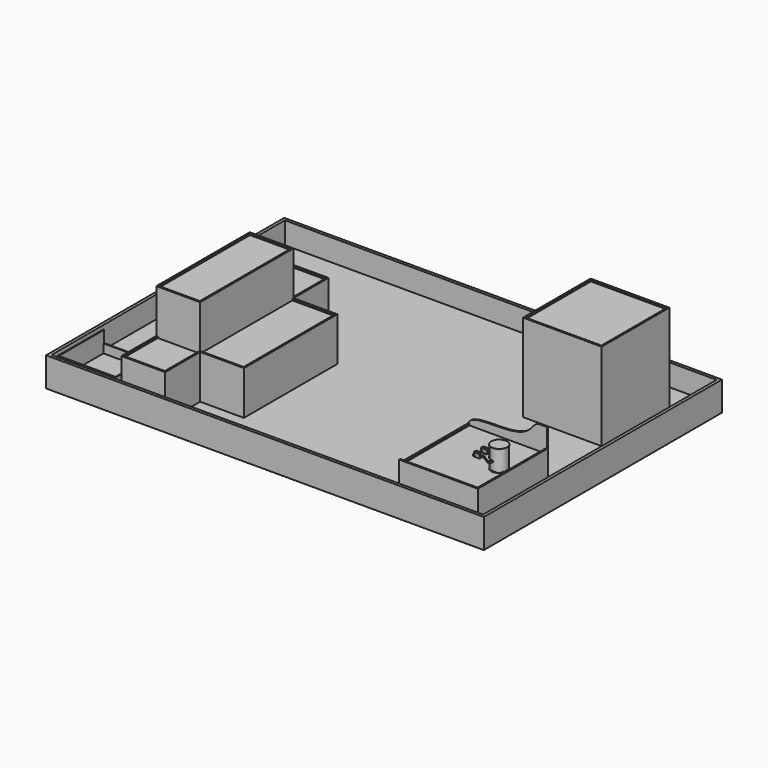
from build123d import *

# Parameters (mm, degrees)
F0_R      = 27.2
F1_DEPTH  = 2.83
F2_R      = 26.4
F3_DEPTH  = 67.36
F4_R      = 27.2
F5_DEPTH  = 2.83
F9_W      = 270
F9_H      = 300
F10_DEPTH = 72
F12_DEPTH = 15
F14_DEPTH = 5
F15_W     = 5
F15_H     = 290
F16_DEPTH = 5
F17_W     = 1500
F17_H     = 1020
F18_DEPTH = 25
F19_W     = 270
F19_H     = 290
F20_DEPTH = 300
F21_W     = 260
F21_H     = 280
F22_DEPTH = 5
F23_W     = 1500
F23_H     = 1020
F23_W_2   = 1480
F23_H_2   = 1000
F24_DEPTH = 75
F26_DEPTH = 150
F27_W     = 150
F27_H     = 400
F28_DEPTH = 150
F29_W     = 140
F29_H     = 390
F30_DEPTH = 5
F31_W     = 140
F31_H     = 145
F31_W_2   = 145
F31_H_2   = 390
F32_DEPTH = 5
F33_R     = 3
F34_DEPTH = 4
F35_R     = 3.99999
F35_2_R   = 3.99999
F36_R     = 3
F37_DEPTH = 8
F38_R     = 3
F39_DEPTH = 8
F40_R     = 3
F40_R_2   = 2.5
F41_DEPTH = 3
F42_R     = 3
F42_R_2   = 2.5
F43_DEPTH = 3
F45_DEPTH = 270.001
F46_W     = 200
F46_H     = 200
F46_W_2   = 194
F46_H_2   = 191
F47_DEPTH = 30
F49_DEPTH = 40
F50_R     = 2.9331626505
F50_R_2   = 2.6879545315
F50_R_3   = 3
F50_R_4   = 2.8111339575
F51_DEPTH = 6


# Not quite as in the source:
# - a fillet or chamfer is up to 0.001 mm smaller than in the source, because OpenCascade refuses the exact size
# - a feature names something its author has since deleted; it is built from what else it names


with BuildPart() as f1:
    # F0 (on Top) → F1 (new body)
    with BuildSketch(Plane.XY):
        Circle(F0_R)
    extrude(amount=F1_DEPTH)

    # F2 (on face) → F3 (join)
    with BuildSketch(Plane.XY.offset(2.83)):
        Circle(F2_R)
    extrude(amount=F3_DEPTH)

    # F4 (on face) → F5 (join)
    with BuildSketch(Plane.XY.offset(70.19)):
        Circle(F4_R)
    extrude(amount=F5_DEPTH)


with BuildPart() as f10:
    # F9 (on Top) → F10 (new body)
    with BuildSketch(Plane.XY):
        with Locations((-87.8, 0)):
            Rectangle(F9_W, F9_H)
    extrude(amount=-F10_DEPTH)

    # F11 (on face) → F12 (join)
    with BuildSketch(Plane.XY):
        Polygon((-222.8, -145), (-222.8, -150), (47.2, -150), (47.2, 150), (42.2, 150), (42.2, -145), align=None)
    extrude(amount=F12_DEPTH)

    # F13 (on face) → F14 (join)
    with BuildSketch(Plane(origin=(0, 150, 0), x_dir=(-1, 0, 0), z_dir=(0, 1, 0))):
        with BuildLine():
            Line((-21.3134280931, 81.3575685024), (-47.2, 81.3575685024))
            Line((-47.2, 81.3575685024), (-47.2, -72))
            Line((-47.2, -72), (222.8, -72))
            Line((222.8, -72), (222.8, 0))
            add(Edge.make_bspline(
                [(-21.3134280931, 81.3575685024), (-6.3059147253, 81.3822787863), (12.9585432644, 38.1268753575), (103.6097013063, 23.6068887567), (223.0224295336, 30.7718731823), (222.8, 0)],
                knots=[0, 0, 0, 0, 0.2487100673, 0.6151112321, 1, 1, 1, 1], degree=3))
        make_face()
    extrude(amount=-F14_DEPTH)

    # F15 (on face) → F16 (join)
    with BuildSketch(Plane.XY):
        with Locations((-220.3, 0)):
            Rectangle(F15_W, F15_H)
    extrude(amount=F16_DEPTH)

    # F17 (on face) → F18 (join)
    with BuildSketch(Plane(origin=(0, 0, -72), x_dir=(1, 0, 0), z_dir=(0, 0, -1))):
        with Locations((-602.8, -260)):
            Rectangle(F17_W, F17_H)
    extrude(amount=F18_DEPTH)

    # F19 (on face) → F20 (join)
    with BuildSketch(Plane.XY.offset(-72)):
        with Locations((-87.8, 525)):
            Rectangle(F19_W, F19_H)
    extrude(amount=F20_DEPTH)

    # F21 (on face) → F22 (cut)
    with BuildSketch(Plane.XY.offset(228)):
        with Locations((-87.8, 525)):
            Rectangle(F21_W, F21_H)
    extrude(amount=-F22_DEPTH, mode=Mode.SUBTRACT)

    # F23 (on face) → F24 (join)
    with BuildSketch(Plane.XY.offset(-72)):
        with Locations((-602.8, 260)):
            Rectangle(F23_W, F23_H)
        with Locations((-602.8, 260)):
            Rectangle(F23_W_2, F23_H_2, mode=Mode.SUBTRACT)
    extrude(amount=F24_DEPTH)

    # F25 (on face) → F26 (join)
    with BuildSketch(Plane.XY.offset(-72)):
        Polygon((-952.8, 460), (-1102.8, 460), (-1102.8, -240), (-952.8, -240), (-952.8, -90), (-802.8, -90), (-802.8, 310), (-952.8, 310), align=None)
    extrude(amount=F26_DEPTH)

    # F27 (on face) → F28 (join)
    with BuildSketch(Plane.XY.offset(78)):
        with Locations((-1027.8, 110)):
            Rectangle(F27_W, F27_H)
    extrude(amount=F28_DEPTH)

    # F29 (on face) → F30 (cut)
    with BuildSketch(Plane.XY.offset(228)):
        with Locations((-1027.8, 110)):
            Rectangle(F29_W, F29_H)
    extrude(amount=-F30_DEPTH, mode=Mode.SUBTRACT)

    # F31 (on face) → F32 (cut)
    with BuildSketch(Plane.XY.offset(78)):
        with Locations((-1027.8, 382.5)):
            Rectangle(F31_W, F31_H)
        with Locations((-880.3, 110)):
            Rectangle(F31_W_2, F31_H_2)
        with Locations((-1027.8, -162.5)):
            Rectangle(F31_W, F31_H)
    extrude(amount=-F32_DEPTH, mode=Mode.SUBTRACT)

    # F46 (on face) → F47 (join)
    with BuildSketch(Plane.XY.offset(-72)):
        with Locations((-1232.8, -130)):
            Rectangle(F46_W, F46_H)
        with Locations((-1232.8, -128.5)):
            Rectangle(F46_W_2, F46_H_2, mode=Mode.SUBTRACT)
    extrude(amount=F47_DEPTH)

    # F48 (on face) → F49 (join)
    with BuildSketch(Plane.XY.offset(-42)):
        Polygon((-1329.8, -30), (-1332.8, -30), (-1332.8, -230), (-1329.8, -230), (-1135.8, -230), (-1132.8, -230), (-1132.8, -30), (-1135.8, -30), (-1135.8, -224), (-1329.8, -224), align=None)
    extrude(amount=F49_DEPTH)


with BuildPart() as f34:
    # F33 (on offset) → F34 (new body, symmetric)
    with BuildSketch(Plane.XY.offset(25)):
        with BuildLine():
            Line((-55, -12), (-74.5, -12))
            Line((-74.5, -12), (-74.5, -13))
            Line((-74.5, -13), (-65.6457513111, -13))
            ThreePointArc((-65.6457513111, -13), (-67, -16), (-65.6457513111, -19))
            Line((-65.6457513111, -19), (-74.5, -19))
            Line((-74.5, -19), (-74.5, -20))
            Line((-74.5, -20), (-55, -20))
            ThreePointArc((-55, -20), (-51, -16), (-55, -12))
        make_face()
        with Locations((-63, -16)):
            Circle(F33_R, mode=Mode.SUBTRACT)
        with Locations((-55, -16)):
            Circle(F33_R, mode=Mode.SUBTRACT)
    extrude(amount=F34_DEPTH, both=True)

    # F35 (radius 4 in the source; OpenCascade refuses exactly that, so slightly less here)
    f35_edges = [f34.edges().sort_by_distance(p)[0] for p in [
        (-74.5, -19.5, 29),
        (-74.5, -12.5, 29),
        (-74.5, -19.5, 21),
        (-74.5, -12.5, 21),
    ]]
    fillet(f35_edges, radius=F35_R)

    # F36 (on face) → F37 (join, through all)
    with BuildSketch(Plane.XZ.offset(20)):
        with Locations((-70.5, 25)):
            Circle(F36_R)
    extrude(amount=-F37_DEPTH)

    # F42 (on offset) → F43 (join, symmetric)
    with BuildSketch(Plane.XY.offset(25)):
        with Locations((-63, -16)):
            Circle(F42_R)
        with Locations((-63, -16)):
            Circle(F42_R_2, mode=Mode.SUBTRACT)
        with Locations((-55, -16)):
            Circle(F42_R)
        with Locations((-55, -16)):
            Circle(F42_R_2, mode=Mode.SUBTRACT)
    extrude(amount=F43_DEPTH, both=True)


with BuildPart() as f34b:
    # F33 (on offset) → F34, piece 2 (new body, symmetric)
    with BuildSketch(Plane.XY.offset(25)):
        with BuildLine():
            Line((-74.5, 13), (-74.5, 12))
            Line((-74.5, 12), (-55, 12))
            ThreePointArc((-55, 12), (-51, 16), (-55, 20))
            Line((-55, 20), (-74.5, 20))
            Line((-74.5, 20), (-74.5, 19))
            Line((-74.5, 19), (-65.6457513111, 19))
            ThreePointArc((-65.6457513111, 19), (-67, 16), (-65.6457513111, 13))
            Line((-65.6457513111, 13), (-74.5, 13))
        make_face()
        with Locations((-63, 16)):
            Circle(F33_R, mode=Mode.SUBTRACT)
        with Locations((-55, 16)):
            Circle(F33_R, mode=Mode.SUBTRACT)
    extrude(amount=F34_DEPTH, both=True)

    # F35#2 (radius 4 in the source; OpenCascade refuses exactly that, so slightly less here)
    f35_2_edges = [f34b.edges().sort_by_distance(p)[0] for p in [
        (-74.5, 12.5, 29),
        (-74.5, 19.5, 29),
        (-74.5, 19.5, 21),
        (-74.5, 12.5, 21),
    ]]
    fillet(f35_2_edges, radius=F35_2_R)

    # F38 (on face) → F39 (join, through all)
    with BuildSketch(Plane(origin=(0, 20, 0), x_dir=(-1, 0, 0), z_dir=(0, 1, 0))):
        with Locations((70.5, 25)):
            Circle(F38_R)
    extrude(amount=-F39_DEPTH)

    # F40 (on offset) → F41 (join, symmetric)
    with BuildSketch(Plane.XY.offset(25)):
        with Locations((-55, 16)):
            Circle(F40_R)
        with Locations((-55, 16)):
            Circle(F40_R_2, mode=Mode.SUBTRACT)
        with Locations((-63, 16)):
            Circle(F40_R)
        with Locations((-63, 16)):
            Circle(F40_R_2, mode=Mode.SUBTRACT)
    extrude(amount=F41_DEPTH, both=True)


with BuildPart() as f45_tool:
    # F44 (on face) → F45 (new body, through all)
    with BuildSketch(Plane(origin=(0, 20, 0), x_dir=(-1, 0, 0), z_dir=(0, 1, 0))):
        with BuildLine():
            Line((71.5, 26), (71.5, 27.2912878475))
            ThreePointArc((71.5, 27.2912878475), (70.5, 27.5), (69.5, 27.2912878475))
            Line((69.5, 27.2912878475), (69.5, 26))
            Line((69.5, 26), (68.2087121525, 26))
            ThreePointArc((68.2087121525, 26), (68, 25), (68.2087121525, 24))
            Line((68.2087121525, 24), (69.5, 24))
            Line((69.5, 24), (69.5, 22.7087121525))
            ThreePointArc((69.5, 22.7087121525), (70.5, 22.5), (71.5, 22.7087121525))
            Line((71.5, 22.7087121525), (71.5, 24))
            Line((71.5, 24), (72.7912878475, 24))
            ThreePointArc((72.7912878475, 24), (73, 25), (72.7912878475, 26))
            Line((72.7912878475, 26), (71.5, 26))
        make_face()
    extrude(amount=-F45_DEPTH)


with BuildPart() as f34_1:
    add(f34.part)

    # F45: cut by f45_tool
    add(f45_tool.part, mode=Mode.SUBTRACT)


with BuildPart() as f34b_1:
    add(f34b.part)

    # F45: cut by f45_tool
    add(f45_tool.part, mode=Mode.SUBTRACT)


with BuildPart() as f51:
    # F50 (on face) → F51 (new body)
    with BuildSketch(Plane.XY.offset(29)):
        with BuildLine():
            ThreePointArc((0.73436121, -28.0007835725), (-28.0000147608, -0.763112347), (-0.7918626795, 27.9992164275))
            Line((-0.7918626795, 27.9992164275), (-5.8697271642, 34.7379657611))
            ThreePointArc((-5.8697271642, 34.7379657611), (-9.0911257385, 36.6690164274), (-12.7480278467, 35.812609736))
            Line((-12.7480278467, 35.812609736), (-33.2897768634, 21.3))
            Line((-33.2897768634, 21.3), (-68.6539217851, 21.3))
            ThreePointArc((-68.6539217851, 21.3), (-70.7752421287, 20.4213203436), (-71.6539217851, 18.3))
            Line((-71.6539217851, 18.3), (-71.6539217851, 13.5))
            ThreePointArc((-71.6539217851, 13.5), (-70.7752421287, 11.3786796564), (-68.6539217851, 10.5))
            Line((-68.6539217851, 10.5), (-38.6539217851, 10.5))
            ThreePointArc((-38.6539217851, 10.5), (-35.1183878792, 9.0355339059), (-33.6539217851, 5.5))
            Line((-33.6539217851, 5.5), (-33.6539217851, -5.5))
            ThreePointArc((-33.6539217851, -5.5), (-35.1183878792, -9.0355339059), (-38.6539217851, -10.5))
            Line((-38.6539217851, -10.5), (-68.6539217851, -10.5))
            ThreePointArc((-68.6539217851, -10.5), (-70.7752421287, -11.3786796564), (-71.6539217851, -13.5))
            Line((-71.6539217851, -13.5), (-71.6539217851, -18.3))
            ThreePointArc((-71.6539217851, -18.3), (-70.7752421287, -20.4213203436), (-68.6539217851, -21.3))
            Line((-68.6539217851, -21.3), (-33.6539217851, -21.3))
            Line((-33.6539217851, -21.3), (-12.3771282772, -35.7756659577))
            ThreePointArc((-12.3771282772, -35.7756659577), (-9.0210911141, -36.6120795445), (-5.9251192441, -35.0701549978))
            Line((-5.9251192441, -35.0701549978), (0.73436121, -28.0007835725))
        make_face()
        with Locations((-62.8900304437, -16)):
            Circle(F50_R, mode=Mode.SUBTRACT)
        with Locations((-55, -16)):
            Circle(F50_R_2, mode=Mode.SUBTRACT)
        with Locations((-63, 16)):
            Circle(F50_R_3, mode=Mode.SUBTRACT)
        with Locations((-55, 16)):
            Circle(F50_R_4, mode=Mode.SUBTRACT)
    extrude(amount=F51_DEPTH)


solid = Compound([f1.part, f10.part, f34_1.part, f34b_1.part, f51.part])
